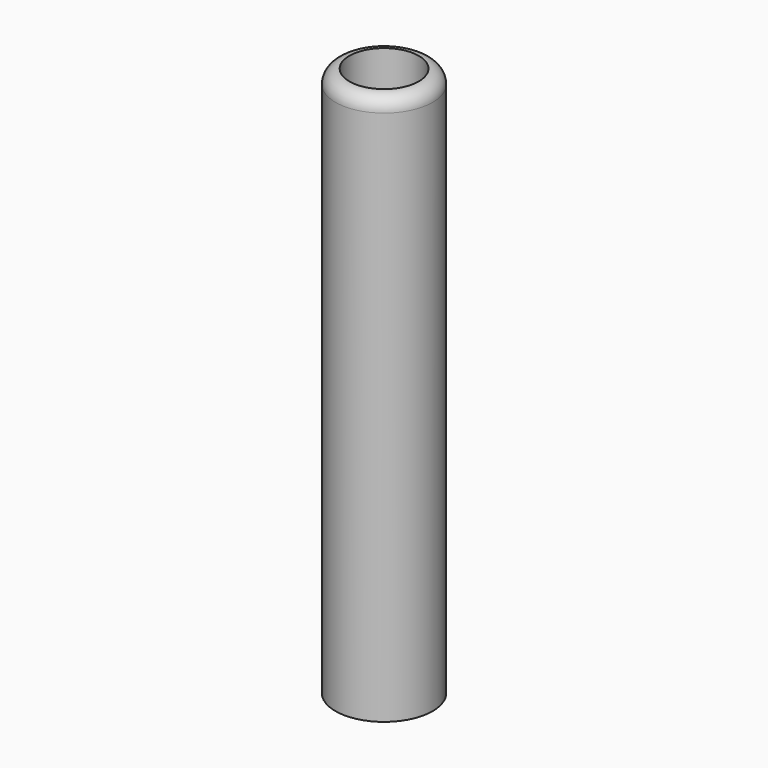
from build123d import *

# Parameters (mm, degrees)
F0_R     = 7
F0_R_2   = 5
F1_DEPTH = 76.2
F0_R_3   = 1.5
F2_DEPTH = 3
F3_R     = 1.99999


# Not quite as in the source:
# - a fillet or chamfer is up to 0.001 mm smaller than in the source, because OpenCascade refuses the exact size


with BuildPart() as f1:
    # F0 (on Top) → F1 (new body)
    with BuildSketch(Plane.XY):
        Circle(F0_R)
        Circle(F0_R_2, mode=Mode.SUBTRACT)
    extrude(amount=F1_DEPTH)

    # F0 (on Top) → F2 (join)
    with BuildSketch(Plane.XY):
        Circle(F0_R)
        Circle(F0_R_2, mode=Mode.SUBTRACT)
        Circle(F0_R_2)
        Circle(F0_R_3, mode=Mode.SUBTRACT)
    extrude(amount=-F2_DEPTH)

    # F3 (radius 2 in the source; OpenCascade refuses exactly that, so slightly less here)
    f3_edges = [f1.edges().sort_by_distance(p)[0] for p in [
        (-7, 0, 76.2),
    ]]
    fillet(f3_edges, radius=F3_R)


solid = f1.part
